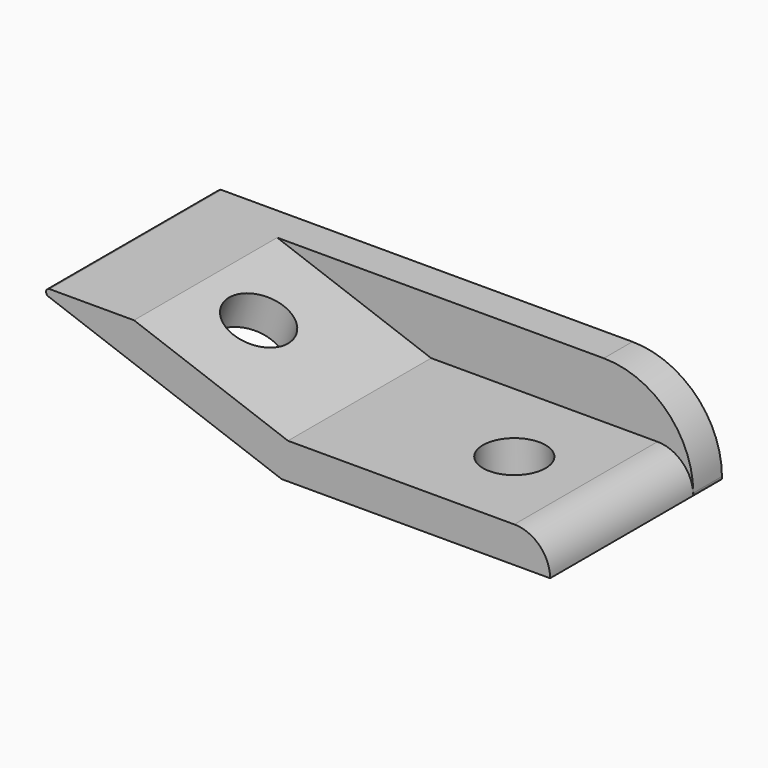
from build123d import *

# Parameters (mm, degrees)
F1_DEPTH    = 2
F3_DEPTH    = 10
F4_T1_DEPTH = 17.6712818196
F5_R        = 1.75
F6_DEPTH    = 2
F7_R        = 1.75
F8_DEPTH    = 2
F9_T1_DEPTH = 15
F9_T6_DEPTH = 20
F9_S7_R     = 5
F9_T8_DEPTH = 12


# Not quite as in the source:
# - a fillet or chamfer that OpenCascade refuses, or shapes differently, is made with other operations: its cross-section is extruded or revolved along the edge and cut away or added


with BuildPart() as f1:
    # F0 (on Front) → F1 (new body)
    with BuildSketch(Plane.XZ):
        with BuildLine():
            Line((-15, 0), (0, 0))
            Line((0, 0), (0, 0.1303021499))
            ThreePointArc((0, 0.1303021499), (-1.4644660941, 3.6658360558), (-5, 5.1303021499))
            Line((-5, 5.1303021499), (-29.0953893118, 5.1303021499))
            Line((-29.0953893118, 5.1303021499), (-15, 0))
        make_face()
    extrude(amount=F1_DEPTH)

    # F2 (on face) → F3 (join)
    with BuildSketch(Plane.XZ.offset(2)):
        Polygon((-23.2477805115, 5.1303021499), (-29.0953893118, 5.1303021499), (-15, 0), (0, 0), (0, 2), (-14.6473460386, 2), align=None)
    extrude(amount=F3_DEPTH)

    # F4: fillet of radius 0.2 on 1 edges, made by hand

    # F4_s2 → F4_t1 (cut)
    with BuildSketch(Plane.XZ.offset(-2.8356409098)):
        with BuildLine():
            ThreePointArc((-27.9611329479, 5.1303021499), (-28.1580944985, 4.9650317854), (-28.0295369765, 4.7423636257))
            Line((-28.0295369765, 4.7423636257), (-29.0953893118, 5.1303021499))
            Line((-29.0953893118, 5.1303021499), (-27.9611329479, 5.1303021499))
        make_face()
    extrude(amount=F4_T1_DEPTH, mode=Mode.SUBTRACT)

    # F5 (on face) → F6 (cut, through all)
    with BuildSketch(Plane(origin=(-1.07062639, 0, -2.9415218311), x_dir=(0.9396926208, 0, -0.3420201433), z_dir=(0.3420201433, 0, 0.9396926208))):
        with Locations((-20.4480432732, -7)):
            Circle(F5_R)
    extrude(amount=-F6_DEPTH, mode=Mode.SUBTRACT)

    # F7 (on face) → F8 (cut, through all)
    with BuildSketch(Plane(origin=(0, 0, 0), x_dir=(1, 0, 0), z_dir=(0, 0, -1))):
        with Locations((-6, 7)):
            Circle(F7_R)
    extrude(amount=-F8_DEPTH, mode=Mode.SUBTRACT)

    # F9: fillet of radius 2 on 1 edges, made by hand

    # F9_s2 → F9_t1 (cut)
    with BuildSketch(Plane.XZ.offset(2)):
        with BuildLine():
            ThreePointArc((0, 0), (-0.5857864376, 1.4142135624), (-2, 2))
            Line((-2, 2), (0, 2))
            Line((0, 2), (0, 0))
        make_face()
    extrude(amount=F9_T1_DEPTH, mode=Mode.SUBTRACT)


with BuildPart() as f9_tool4:
    # F9_s5 → F9_t6 (new body)
    with BuildSketch(Plane.XZ.offset(-3)):
        with BuildLine():
            ThreePointArc((0, 0), (-0.5857864376, 1.4142135624), (-2, 2))
            Line((-2, 2), (0, 2))
            Line((0, 2), (0, 0))
        make_face()
    extrude(amount=F9_T6_DEPTH)

    # F9_s7 → F9_t8 (cut, symmetric)
    with BuildSketch(Plane.XZ.offset(7)):
        with Locations((-5, 0.1303021499)):
            Circle(F9_S7_R)
    extrude(amount=F9_T8_DEPTH, both=True, mode=Mode.SUBTRACT)


with BuildPart() as f1_1:
    add(f1.part)

    # F9_t3: cut F9_tool4
    add(f9_tool4.part, mode=Mode.SUBTRACT)


solid = f1_1.part
